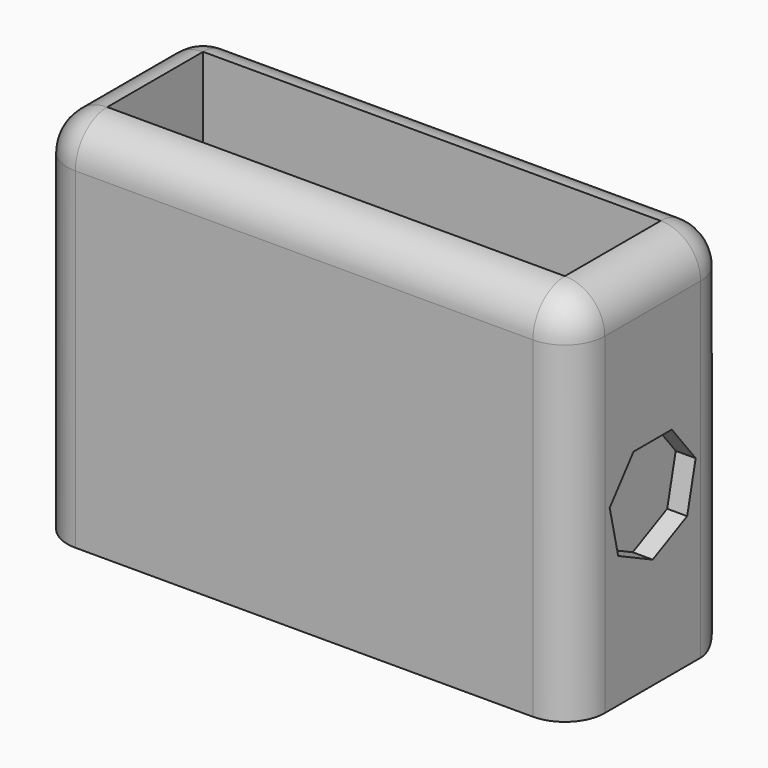
from build123d import *

# Parameters (mm, degrees)
F0_W         = 68.380638957
F0_H         = 47.2927317023
F1_DEPTH     = 25.4
F2_R         = 5.08
F3_TEXT_SIZE = 14.8987260563
F4_DEPTH     = 5.08
F6_DEPTH     = 38.1
F8_DEPTH     = 2.54
F10_DEPTH    = 2.54


# Not quite as in the source:
# - Text() gives the source's letters only with a copy of the font that has no kerning and outlines rounded to 1/6400 em; it was checked with that copy


with BuildPart() as f1:
    # F0 (on Front) → F1 (new body)
    with BuildSketch(Plane.XZ):
        with Locations((34.1903194785, 23.6463658512)):
            Rectangle(F0_W, F0_H)
    extrude(amount=F1_DEPTH)

    # F2
    f2_edges = [f1.edges().sort_by_distance(p)[0] for p in [
        (34.190319, -25.4, 47.292732),
        (68.380639, -25.4, 23.646366),
        (68.380639, -12.7, 47.292732),
        (68.380639, 0, 23.646366),
        (0, -25.4, 23.646366),
        (0, 0, 23.646366),
        (34.190319, 0, 0),
        (34.190319, 0, 47.292732),
        (0, -12.7, 47.292732),
    ]]
    fillet(f2_edges, radius=F2_R)

    # F3 (on face) → F4 (join)
    with BuildSketch(Plane(origin=(0, 0, 0), x_dir=(-1, 0, 0), z_dir=(0, 1, 0))):
        with Locations((-57.5769837321, 18.0941467093)):
            Text('Celeste', F3_TEXT_SIZE, font='Open Sans', text_align=(TextAlign.LEFT, TextAlign.BOTTOM))
    extrude(amount=F4_DEPTH)

    # F5 (on face) → F6 (cut)
    with BuildSketch(Plane.XY.offset(47.2927317023)):
        Polygon((5.08, -20.32), (63.300638957, -20.32), (63.300638957, -5.8012120426), (63.300638957, -5.08), (5.08, -5.08), (5.08, -5.8012120426), align=None)
    extrude(amount=-F6_DEPTH, mode=Mode.SUBTRACT)

    # F7 (on face) → F8 (cut)
    with BuildSketch(Plane(origin=(0, 0, 0), x_dir=(0, -1, 0), z_dir=(-1, 0, 0))):
        Polygon((12.7, 27.4299317023), (12.7, 13.660592899), (18.3630609533, 16.3877793188), (19.7617215033, 22.5157115798), (15.8427617285, 27.4299317023), align=None)
        Polygon((7.0369390467, 16.3877793188), (12.7, 13.660592899), (12.7, 27.4299317023), (9.5572382715, 27.4299317023), (5.6382784967, 22.5157115798), align=None)
    extrude(amount=-F8_DEPTH, mode=Mode.SUBTRACT)

    # F9 (on face) → F10 (cut)
    with BuildSketch(Plane.YZ.offset(68.380638957)):
        Polygon((-18.184644365, 16.7325079226), (-12.7, 14.0912424032), (-12.7, 27.4267736822), (-15.743747992, 27.4267736822), (-19.5392396568, 22.6673776726), align=None)
        Polygon((-12.7, 27.4267736822), (-12.7, 14.0912424032), (-7.215355635, 16.7325079226), (-5.8607603432, 22.6673776726), (-9.656252008, 27.4267736822), align=None)
    extrude(amount=-F10_DEPTH, mode=Mode.SUBTRACT)


solid = f1.part
